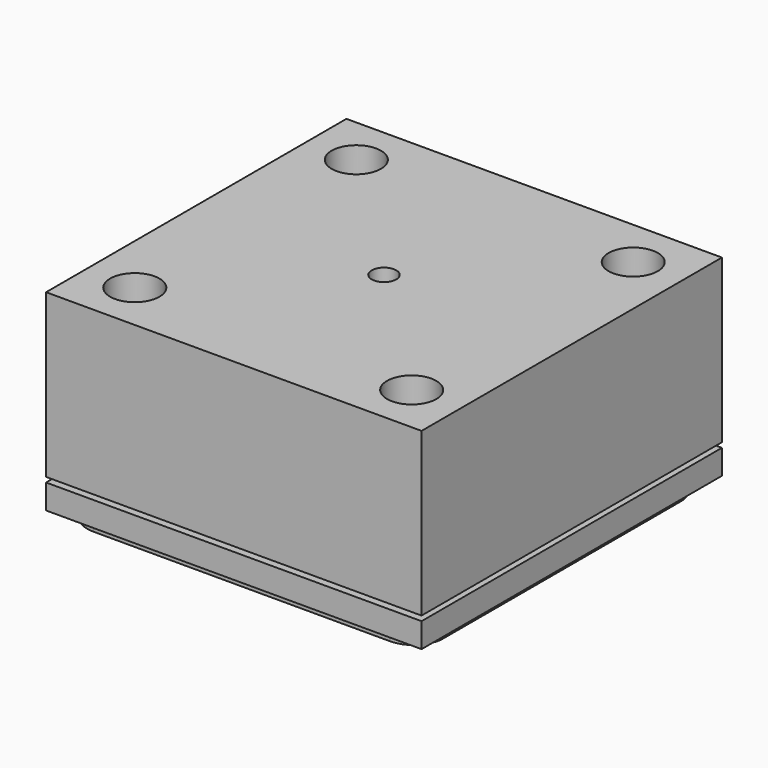
from build123d import *

# Parameters (mm, degrees)
F0_W      = 72.2
F0_H      = 72.2
F1_DEPTH  = 2
F2_R      = 6
F3_R      = 3.175
F3_R_2    = 2
F4_DEPTH  = 2.001
F5_R      = 5
F5_R_2    = 3.175
F5_W      = 20
F5_H      = 20
F5_R_3    = 2
F6_DEPTH  = 1
F8_W      = 76.2
F8_H      = 76.2
F9_DEPTH  = 5
F10_R     = 0.1
F10_R_2   = 3.175
F11_DEPTH = 7.001
F10_R_3   = 1
F12_DEPTH = 4
F10_R_4   = 19.3
F10_R_5   = 15.6
F13_DEPTH = 3
F15_W     = 72.2
F15_H     = 72.2
F16_DEPTH = 1
F17_R     = 3.175
F17_R_2   = 2
F18_DEPTH = 8.001
F19_R     = 6
F21_W     = 76.2
F21_H     = 76.2
F22_DEPTH = 33
F23_R     = 3.175
F23_R_2   = 2.5
F24_DEPTH = 41.001
F23_R_3   = 5
F25_DEPTH = 11
F26_R     = 3.175
F27_DEPTH = 20
F26_R_2   = 19.3
F26_R_3   = 15.6
F28_DEPTH = 2
F26_R_4   = 12
F26_R_5   = 2.5
F29_DEPTH = 28


with BuildPart() as f1:
    # F0 (on Top) → F1 (new body)
    with BuildSketch(Plane.XY):
        Rectangle(F0_W, F0_H)
    extrude(amount=F1_DEPTH)

    # F2
    f2_edges = [f1.edges().sort_by_distance(p)[0] for p in [
        (-36.1, -36.1, 1),
        (36.1, -36.1, 1),
        (-36.1, 36.1, 1),
        (36.1, 36.1, 1),
    ]]
    fillet(f2_edges, radius=F2_R)

    # F3 (on face) → F4 (cut, through all)
    with BuildSketch(Plane.XY.offset(2)):
        with Locations((-28.1, 28.1)):
            Circle(F3_R)
        with Locations((-10.1, 25.1)):
            Circle(F3_R)
        with Locations((10.1, 25.1)):
            Circle(F3_R)
        with Locations((28.1, 28.1)):
            Circle(F3_R)
        with Locations((-25.1, 10.1)):
            Circle(F3_R)
        with Locations((-5, 5)):
            Circle(F3_R_2)
        with Locations((5, 5)):
            Circle(F3_R_2)
        with Locations((25.1, 10.1)):
            Circle(F3_R)
        with Locations((25.1, -10.1)):
            Circle(F3_R)
        with Locations((5, -5)):
            Circle(F3_R_2)
        with Locations((-5, -5)):
            Circle(F3_R_2)
        with Locations((-25.1, -10.1)):
            Circle(F3_R)
        with Locations((-28.1, -28.1)):
            Circle(F3_R)
        with Locations((-10.1, -25.1)):
            Circle(F3_R)
        with BuildLine():
            ThreePointArc((13.275, -25.1), (10.1, -21.925), (6.925, -25.1))
            ThreePointArc((6.925, -25.1), (10.1, -28.275), (13.275, -25.1))
        make_face()
        with Locations((28.1, -28.1)):
            Circle(F3_R)
    extrude(amount=-F4_DEPTH, mode=Mode.SUBTRACT)

    # F5 (on face) → F6 (cut)
    with BuildSketch(Plane(origin=(0, 0, 0), x_dir=(1, 0, 0), z_dir=(0, 0, -1))):
        with Locations((-10.1, 25.1)):
            Circle(F5_R)
        with Locations((-10.1, 25.1)):
            Circle(F5_R_2, mode=Mode.SUBTRACT)
        with Locations((10.1, 25.1)):
            Circle(F5_R)
        with Locations((10.1, 25.1)):
            Circle(F5_R_2, mode=Mode.SUBTRACT)
        with Locations((25.1, 10.1)):
            Circle(F5_R)
        with Locations((25.1, 10.1)):
            Circle(F5_R_2, mode=Mode.SUBTRACT)
        with Locations((-25.1, 10.1)):
            Circle(F5_R)
        with Locations((-25.1, 10.1)):
            Circle(F5_R_2, mode=Mode.SUBTRACT)
        Rectangle(F5_W, F5_H)
        with Locations((-5, -5)):
            Circle(F5_R_3, mode=Mode.SUBTRACT)
        with Locations((5, -5)):
            Circle(F5_R_3, mode=Mode.SUBTRACT)
        with Locations((-5, 5)):
            Circle(F5_R_3, mode=Mode.SUBTRACT)
        with Locations((5, 5)):
            Circle(F5_R_3, mode=Mode.SUBTRACT)
        with Locations((-25.1, -10.1)):
            Circle(F5_R)
        with Locations((-25.1, -10.1)):
            Circle(F5_R_2, mode=Mode.SUBTRACT)
        with Locations((-10.1, -25.1)):
            Circle(F5_R)
        with Locations((-10.1, -25.1)):
            Circle(F5_R_2, mode=Mode.SUBTRACT)
        with Locations((10.1, -25.1)):
            Circle(F5_R)
        with Locations((10.1, -25.1)):
            Circle(F5_R_2, mode=Mode.SUBTRACT)
        with Locations((25.1, -10.1)):
            Circle(F5_R)
        with Locations((25.1, -10.1)):
            Circle(F5_R_2, mode=Mode.SUBTRACT)
    extrude(amount=-F6_DEPTH, mode=Mode.SUBTRACT)


with BuildPart() as f9:
    # F8 (on offset) → F9 (new body)
    with BuildSketch(Plane.XY.offset(2)):
        Rectangle(F8_W, F8_H)
    extrude(amount=F9_DEPTH)

    # F10 (on face) → F11 (cut, through all)
    with BuildSketch(Plane.XY.offset(7)):
        with Locations((-5, 5)):
            Circle(F10_R)
        with Locations((-5, -5)):
            Circle(F10_R)
        with Locations((5, -5)):
            Circle(F10_R)
        with Locations((5, 5)):
            Circle(F10_R)
        with Locations((-28.1, 28.1)):
            Circle(F10_R_2)
        with Locations((-10.1, 25.1)):
            Circle(F10_R_2)
        with Locations((10.1, 25.1)):
            Circle(F10_R_2)
        with Locations((28.1, 28.1)):
            Circle(F10_R_2)
        with Locations((25.1, 10.1)):
            Circle(F10_R_2)
        with Locations((25.1, -10.1)):
            Circle(F10_R_2)
        with Locations((28.1, -28.1)):
            Circle(F10_R_2)
        with Locations((10.1, -25.1)):
            Circle(F10_R_2)
        with Locations((-10.1, -25.1)):
            Circle(F10_R_2)
        with Locations((-28.1, -28.1)):
            Circle(F10_R_2)
        with Locations((-25.1, -10.1)):
            Circle(F10_R_2)
        with Locations((-25.1, 10.1)):
            Circle(F10_R_2)
    extrude(amount=-F11_DEPTH, mode=Mode.SUBTRACT)

    # F10 (on face) → F12 (cut)
    with BuildSketch(Plane.XY.offset(7)):
        with Locations((-5, 5)):
            Circle(F10_R_3)
        with Locations((-5, 5)):
            Circle(F10_R, mode=Mode.SUBTRACT)
        with Locations((5, 5)):
            Circle(F10_R_3)
        with Locations((5, 5)):
            Circle(F10_R, mode=Mode.SUBTRACT)
        with Locations((5, -5)):
            Circle(F10_R_3)
        with Locations((5, -5)):
            Circle(F10_R, mode=Mode.SUBTRACT)
        with Locations((-5, -5)):
            Circle(F10_R_3)
        with Locations((-5, -5)):
            Circle(F10_R, mode=Mode.SUBTRACT)
    extrude(amount=-F12_DEPTH, mode=Mode.SUBTRACT)

    # F10 (on face) → F13 (cut)
    with BuildSketch(Plane.XY.offset(7)):
        Circle(F10_R_4)
        Circle(F10_R_5, mode=Mode.SUBTRACT)
    extrude(amount=-F13_DEPTH, mode=Mode.SUBTRACT)


with BuildPart() as f16:
    # F15 (on offset) → F16 (new body)
    with BuildSketch(Plane.XY.offset(7)):
        Rectangle(F15_W, F15_H)
    extrude(amount=F16_DEPTH)

    # F17 (on face) → F18 (cut, through all)
    with BuildSketch(Plane.XY.offset(8)):
        with Locations((-10.1, 25.1)):
            Circle(F17_R)
        with Locations((-25.1, 10.1)):
            Circle(F17_R)
        with Locations((-5, -5)):
            Circle(F17_R_2)
        with Locations((25.1, -10.1)):
            Circle(F17_R)
        with Locations((-10.1, -25.1)):
            Circle(F17_R)
        with Locations((-28.1, 28.1)):
            Circle(F17_R)
        with Locations((10.1, 25.1)):
            Circle(F17_R)
        with Locations((28.1, 28.1)):
            Circle(F17_R)
        with Locations((25.1, 10.1)):
            Circle(F17_R)
        with Locations((5, 5)):
            Circle(F17_R_2)
        with Locations((-5, 5)):
            Circle(F17_R_2)
        with Locations((5, -5)):
            Circle(F17_R_2)
        with Locations((10.1, -25.1)):
            Circle(F17_R)
        with Locations((28.1, -28.1)):
            Circle(F17_R)
        with Locations((-28.1, -28.1)):
            Circle(F17_R)
        with Locations((-25.1, -10.1)):
            Circle(F17_R)
    extrude(amount=-F18_DEPTH, mode=Mode.SUBTRACT)

    # F19
    f19_edges = [f16.edges().sort_by_distance(p)[0] for p in [
        (-36.1, -36.1, 7.5),
        (36.1, -36.1, 7.5),
        (36.1, 36.1, 7.5),
        (-36.1, 36.1, 7.5),
    ]]
    fillet(f19_edges, radius=F19_R)


with BuildPart() as f22:
    # F21 (on offset) → F22 (new body)
    with BuildSketch(Plane.XY.offset(8)):
        Rectangle(F21_W, F21_H)
    extrude(amount=F22_DEPTH)

    # F23 (on face) → F24 (cut, through all)
    with BuildSketch(Plane.XY.offset(41)):
        with Locations((-28.1, 28.1)):
            Circle(F23_R)
        with Locations((28.1, 28.1)):
            Circle(F23_R)
        Circle(F23_R_2)
        with Locations((-28.1, -28.1)):
            Circle(F23_R)
        with Locations((28.1, -28.1)):
            Circle(F23_R)
    extrude(amount=-F24_DEPTH, mode=Mode.SUBTRACT)

    # F23 (on face) → F25 (cut)
    with BuildSketch(Plane.XY.offset(41)):
        with Locations((-28.1, 28.1)):
            Circle(F23_R_3)
        with Locations((-28.1, 28.1)):
            Circle(F23_R, mode=Mode.SUBTRACT)
        with Locations((28.1, 28.1)):
            Circle(F23_R_3)
        with Locations((28.1, 28.1)):
            Circle(F23_R, mode=Mode.SUBTRACT)
        with Locations((28.1, -28.1)):
            Circle(F23_R_3)
        with Locations((28.1, -28.1)):
            Circle(F23_R, mode=Mode.SUBTRACT)
        with Locations((-28.1, -28.1)):
            Circle(F23_R_3)
        with Locations((-28.1, -28.1)):
            Circle(F23_R, mode=Mode.SUBTRACT)
    extrude(amount=-F25_DEPTH, mode=Mode.SUBTRACT)

    # F26 (on face) → F27 (cut)
    with BuildSketch(Plane(origin=(0, 0, 8), x_dir=(1, 0, 0), z_dir=(0, 0, -1))):
        with Locations((-10.1, 25.1)):
            Circle(F26_R)
        with Locations((10.1, 25.1)):
            Circle(F26_R)
        with Locations((25.1, 10.1)):
            Circle(F26_R)
        with Locations((25.1, -10.1)):
            Circle(F26_R)
        with Locations((10.1, -25.1)):
            Circle(F26_R)
        with Locations((-10.1, -25.1)):
            Circle(F26_R)
        with Locations((-25.1, -10.1)):
            Circle(F26_R)
        with Locations((-25.1, 10.1)):
            Circle(F26_R)
    extrude(amount=-F27_DEPTH, mode=Mode.SUBTRACT)

    # F26 (on face) → F28 (cut)
    with BuildSketch(Plane(origin=(0, 0, 8), x_dir=(1, 0, 0), z_dir=(0, 0, -1))):
        Circle(F26_R_2)
        Circle(F26_R_3, mode=Mode.SUBTRACT)
    extrude(amount=-F28_DEPTH, mode=Mode.SUBTRACT)

    # F26 (on face) → F29 (cut)
    with BuildSketch(Plane(origin=(0, 0, 8), x_dir=(1, 0, 0), z_dir=(0, 0, -1))):
        Circle(F26_R_4)
        Circle(F26_R_5, mode=Mode.SUBTRACT)
    extrude(amount=-F29_DEPTH, mode=Mode.SUBTRACT)


solid = Compound([f1.part, f9.part, f16.part, f22.part])
